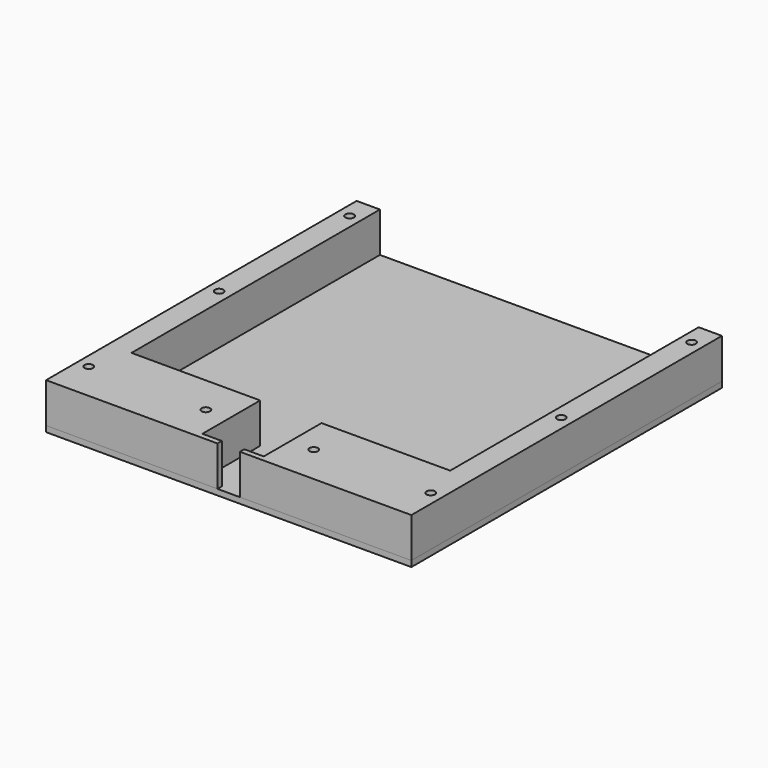
from build123d import *

# Parameters (mm, degrees)
F0_W     = 6
F0_H     = 80
F0_W_2   = 5
F0_H_2   = 1.4
F1_DEPTH = 10.3
F0_W_3   = 5.8
F2_DEPTH = 1.5
F3_D     = 2.2
F3_2_D   = 2.2


with BuildPart() as f1:
    # F0 (on Top) → F1 (new body)
    with BuildSketch(Plane.XY):
        with Locations((-3, 40)):
            Rectangle(F0_W, F0_H)
        Polygon((33.15, 0), (0, 0), (-6, 0), (-6, -20), (33.15, -20), (33.15, -18.6), align=None)
        with Locations((35.65, -19.3)):
            Rectangle(F0_W_2, F0_H_2)
    extrude(amount=F1_DEPTH)

    # F3 (through all)
    with Locations(Plane(origin=(0, 0, 0), x_dir=(1, 0, 0), z_dir=(0, 0, -1))):
        with Locations((-3, -74), (85.1, -74), (85.1, -32), (-3, -32), (-3, 10), (27.15, 10), (54.95, 10), (85.1, 10)):
            Hole(F3_D / 2)


with BuildPart() as f1b:
    # F0 (on Top) → F1, piece 2 (new body)
    with BuildSketch(Plane.XY):
        Polygon((82.1, 0), (48.95, 0), (48.95, -18.6), (48.95, -20), (88.1, -20), (88.1, 0), align=None)
        with Locations((85.1, 40)):
            Rectangle(F0_W, F0_H)
        with Locations((46.45, -19.3)):
            Rectangle(F0_W_2, F0_H_2)
    extrude(amount=F1_DEPTH)

    # F3#2 (through all)
    with Locations(Plane(origin=(0, 0, 0), x_dir=(1, 0, 0), z_dir=(0, 0, -1))):
        with Locations((-3, -74), (85.1, -74), (85.1, -32), (-3, -32), (-3, 10), (27.15, 10), (54.95, 10), (85.1, 10)):
            Hole(F3_2_D / 2)


with BuildPart() as f2:
    # F0 (on Top) → F2 (new body)
    with BuildSketch(Plane.XY):
        Polygon((0, 80), (0, 0), (33.15, 0), (48.95, 0), (82.1, 0), (82.1, 80), align=None)
        with Locations((-3, 40)):
            Rectangle(F0_W, F0_H)
        Polygon((33.15, 0), (0, 0), (-6, 0), (-6, -20), (33.15, -20), (33.15, -18.6), align=None)
        Polygon((82.1, 0), (48.95, 0), (48.95, -18.6), (48.95, -20), (88.1, -20), (88.1, 0), align=None)
        with Locations((35.65, -19.3)):
            Rectangle(F0_W_2, F0_H_2)
        with Locations((85.1, 40)):
            Rectangle(F0_W, F0_H)
        with Locations((46.45, -19.3)):
            Rectangle(F0_W_2, F0_H_2)
        with Locations((41.05, -19.3)):
            Rectangle(F0_W_3, F0_H_2)
        Polygon((48.95, 0), (33.15, 0), (33.15, -18.6), (38.15, -18.6), (43.95, -18.6), (48.95, -18.6), align=None)
    extrude(amount=-F2_DEPTH)


solid = Compound([f1.part, f1b.part, f2.part])
